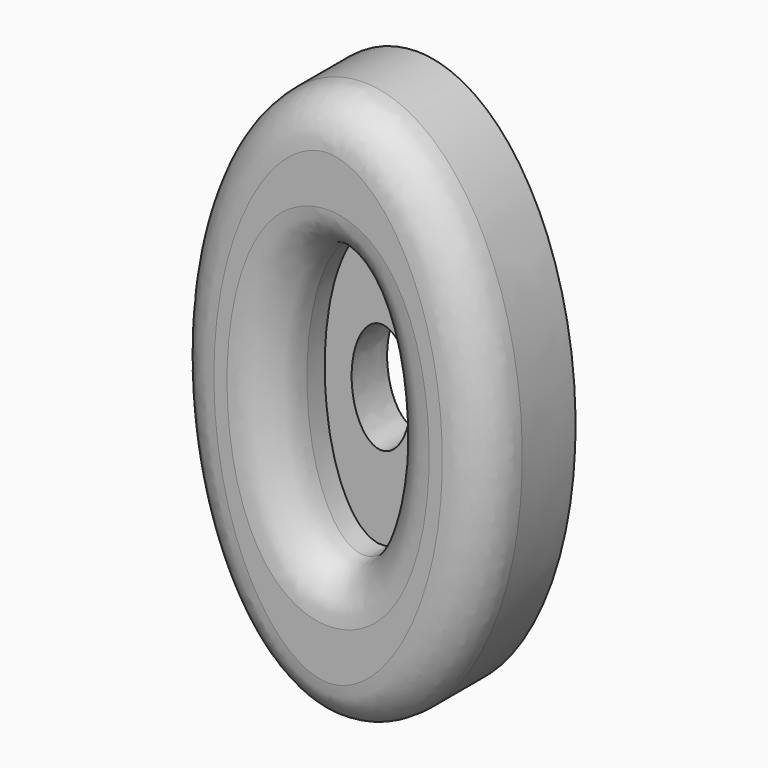
from build123d import *

# Parameters (mm, degrees)
F1_DEPTH = 12.7
F2_DEPTH = 5.08
F3_R     = 5.08


with BuildPart() as f1:
    # F0 (on Front) → F1 (new body)
    with BuildSketch(Plane.XZ):
        with BuildLine():
            add(Edge.make_bspline(
                [(0, 31.75), (-31.4346147509, 31.75), (-15.7173073754, -15.875), (0, -63.5), (15.7173073754, -15.875), (31.4346147509, 31.75), (0, 31.75)],
                knots=[0, 0, 0, 2.0943951024, 2.0943951024, 4.1887902048, 4.1887902048, 6.2831853072, 6.2831853072, 6.2831853072], degree=2, weights=[1, 0.5, 1, 0.5, 1, 0.5, 1]))
        make_face()
        with BuildLine():
            add(Edge.make_bspline(
                [(0, 15.875), (-11.2377592119, 15.875), (-5.6188796059, -7.9375), (0, -31.75), (5.6188796059, -7.9375), (11.2377592119, 15.875), (0, 15.875)],
                knots=[0, 0, 0, 2.0943951024, 2.0943951024, 4.1887902048, 4.1887902048, 6.2831853072, 6.2831853072, 6.2831853072], degree=2, weights=[1, 0.5, 1, 0.5, 1, 0.5, 1]))
        make_face(mode=Mode.SUBTRACT)
    extrude(amount=F1_DEPTH)

    # F3
    f3_edges = [f1.edges().sort_by_distance(p)[0] for p in [
        (-1e-06, -12.7, -31.75),
        (-1.7e-05, -12.7, -15.875),
    ]]
    fillet(f3_edges, radius=F3_R)


with BuildPart() as f2:
    # F0 (on Front) → F2 (new body)
    with BuildSketch(Plane.XZ):
        with BuildLine():
            add(Edge.make_bspline(
                [(0, 15.875), (-11.2377592119, 15.875), (-5.6188796059, -7.9375), (0, -31.75), (5.6188796059, -7.9375), (11.2377592119, 15.875), (0, 15.875)],
                knots=[0, 0, 0, 2.0943951024, 2.0943951024, 4.1887902048, 4.1887902048, 6.2831853072, 6.2831853072, 6.2831853072], degree=2, weights=[1, 0.5, 1, 0.5, 1, 0.5, 1]))
        make_face()
        with BuildLine():
            add(Edge.make_bspline(
                [(0, 6.35), (-5.8951377227, 6.35), (-2.9475688614, -3.175), (0, -12.7), (2.9475688614, -3.175), (5.8951377227, 6.35), (0, 6.35)],
                knots=[0, 0, 0, 2.0943951024, 2.0943951024, 4.1887902048, 4.1887902048, 6.2831853072, 6.2831853072, 6.2831853072], degree=2, weights=[1, 0.5, 1, 0.5, 1, 0.5, 1]))
        make_face(mode=Mode.SUBTRACT)
    extrude(amount=F2_DEPTH)


solid = Compound([f1.part, f2.part])
